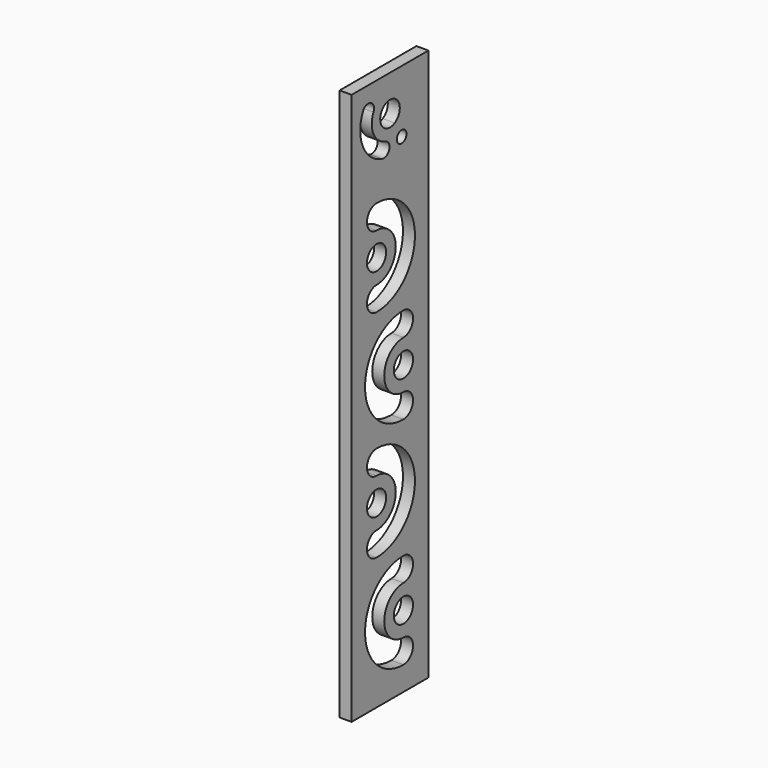
from build123d import *

# Parameters (mm, degrees)
F0_W      = 63.5
F0_H      = 63.5
F0_W_2    = 50.8
F0_H_2    = 50.8
F1_DEPTH  = 165.1
F3_R      = 6.477
F4_DEPTH  = 25.4
F6_DEPTH  = 25.4
F7_R      = 6.35
F8_DEPTH  = 63.501
F9_W      = 145.7979530096
F9_H      = 377.9422044754
F9_W_2    = 50.8
F9_H_2    = 292.1
F10_DEPTH = 63.5
F11_W     = 97.6704657078
F11_H     = 338.8985395432
F12_DEPTH = 57.151


# Not quite as in the source:
# - ends of sketch curves that miss each other by under 0.0002 mm in the source are joined


with BuildPart() as f1:
    # F0 (on Top) → F1 (new body, symmetric)
    with BuildSketch(Plane.XY):
        Rectangle(F0_W, F0_H)
        Rectangle(F0_W_2, F0_H_2, mode=Mode.SUBTRACT)
    extrude(amount=F1_DEPTH, both=True)

    # F3 (on face) → F4 (cut)
    with BuildSketch(Plane.YZ.offset(31.75)):
        with Locations((0, 146.05)):
            Circle(F3_R)
        with BuildLine():
            ThreePointArc((10.1385245046, 129.1766616857), (14.6288058895, 132.8781640138), (17.8406687878, 137.7307595176))
            ThreePointArc((17.8406687878, 137.7307595176), (19.4934269332, 143.3103775076), (19.4426449846, 149.1294124443))
            ThreePointArc((19.4426449846, 149.1294124443), (15.0835370951, 152.2964897102), (11.9164598293, 147.9373818207))
            ThreePointArc((11.9164598293, 147.9373818207), (11.9475842494, 144.3708765369), (10.9346034506, 140.9511106721))
            ThreePointArc((10.9346034506, 140.9511106721), (8.9660423194, 137.9769392343), (6.2139343738, 135.708276517))
            ThreePointArc((6.2139343738, 135.708276517), (4.9104220235, 130.4801740359), (10.1385245046, 129.1766616857))
        make_face()
        with BuildLine():
            ThreePointArc((-10.1385245046, 129.1766616857), (-4.9104220235, 130.4801740359), (-6.2139343738, 135.708276517))
            ThreePointArc((-6.2139343738, 135.708276517), (-8.9660423194, 137.9769392343), (-10.9346034506, 140.9511106721))
            ThreePointArc((-10.9346034506, 140.9511106721), (-11.9475842494, 144.3708765369), (-11.9164598293, 147.9373818207))
            ThreePointArc((-11.9164598293, 147.9373818207), (-15.0835370951, 152.2964897102), (-19.4426449846, 149.1294124443))
            ThreePointArc((-19.4426449846, 149.1294124443), (-19.4934269332, 143.3103775076), (-17.8406687878, 137.7307595176))
            ThreePointArc((-17.8406687878, 137.7307595176), (-14.6288058895, 132.8781640138), (-10.1385245046, 129.1766616857))
        make_face()
    extrude(amount=-F4_DEPTH, mode=Mode.SUBTRACT)

    # F5 (on face) → F6 (cut)
    with BuildSketch(Plane(origin=(-31.75, 0, 0), x_dir=(0, -1, 0), z_dir=(-1, 0, 0))):
        with BuildLine():
            ThreePointArc((-3.1401119103, 140.3850881569), (3.2873259769, 140.4692279278), (6.477, 146.05))
            ThreePointArc((6.477, 146.05), (-3.2873259769, 151.6307720722), (-3.1401119103, 140.3850881569))
        make_face()
        with BuildLine():
            ThreePointArc((-4.5213527214, 132.1654121492), (-4.960680137, 133.7768464516), (-6.1570821771, 134.9423297193))
            ThreePointArc((-6.1570821771, 134.9423297193), (-10.4320253058, 130.5539778468), (-4.5213527214, 132.1654121492))
        make_face()
        with BuildLine():
            ThreePointArc((3.1226517792, 134.3961049058), (0.4285749428, 129.7298269458), (5.0948529028, 127.0357501095))
            ThreePointArc((5.0948529028, 127.0357501095), (17.8406687878, 137.7307595176), (17.8406687878, 154.3692404824))
            ThreePointArc((17.8406687878, 154.3692404824), (12.777460542, 156.2120975737), (10.9346034506, 151.1488893279))
            ThreePointArc((10.9346034506, 151.1488893279), (10.9346034506, 140.9511106721), (3.1226517792, 134.3961049058))
        make_face()
    extrude(amount=-F6_DEPTH, mode=Mode.SUBTRACT)

    # F7 (on face) → F8 (cut, through all)
    with BuildSketch(Plane.YZ.offset(31.75)):
        with BuildLine():
            ThreePointArc((-8.89, 107.949999693), (-15.239999693, 101.6), (-8.89, 95.250000307))
            ThreePointArc((-8.89, 95.250000307), (3.81, 82.55), (-8.89, 69.85))
            ThreePointArc((-8.89, 69.85), (-15.239999693, 63.5), (-8.89, 57.150000307))
            ThreePointArc((-8.89, 57.150000307), (16.509999693, 82.55), (-8.89, 107.949999693))
        make_face()
        with BuildLine():
            ThreePointArc((8.89, 3.07e-07), (15.239999693, 6.35), (8.89, 12.699999693))
            ThreePointArc((8.89, 12.699999693), (-3.81, 25.4), (8.89, 38.1))
            ThreePointArc((8.89, 38.1), (15.24, 44.45), (8.89, 50.8))
            ThreePointArc((8.89, 50.8), (-16.509999693, 25.4), (8.89, 3.07e-07))
        make_face()
        with BuildLine():
            ThreePointArc((-8.89, -6.350000307), (-15.239999693, -12.7), (-8.89, -19.049999693))
            ThreePointArc((-8.89, -19.049999693), (3.81, -31.75), (-8.89, -44.45))
            ThreePointArc((-8.89, -44.45), (-15.239999693, -50.8), (-8.89, -57.149999693))
            ThreePointArc((-8.89, -57.149999693), (16.509999693, -31.75), (-8.89, -6.350000307))
        make_face()
        with BuildLine():
            ThreePointArc((8.89, -114.299999693), (15.239999693, -107.95), (8.89, -101.600000307))
            ThreePointArc((8.89, -101.600000307), (-3.81, -88.9), (8.89, -76.2))
            ThreePointArc((8.89, -76.2), (15.24, -69.85), (8.89, -63.5))
            ThreePointArc((8.89, -63.5), (-16.509999693, -88.9), (8.89, -114.299999693))
        make_face()
        with Locations((-8.89, 82.55)):
            Circle(F7_R)
        with Locations((8.89, 25.4)):
            Circle(F7_R)
        with Locations((8.89, -88.9)):
            Circle(F7_R)
        with Locations((-8.89, -31.75)):
            Circle(F7_R)
    extrude(amount=-F8_DEPTH, mode=Mode.SUBTRACT)

    # F9 (on face) → F10 (cut, symmetric)
    with BuildSketch(Plane(origin=(25.4, 0, 0), x_dir=(0, -1, 0), z_dir=(-1, 0, 0))):
        Rectangle(F9_W, F9_H)
        with Locations((0, 19.05)):
            Rectangle(F9_W_2, F9_H_2, mode=Mode.SUBTRACT)
    extrude(amount=F10_DEPTH, both=True, mode=Mode.SUBTRACT)

    # F11 (on face) → F12 (cut, through all)
    with BuildSketch(Plane.YZ.offset(-25.4)):
        Rectangle(F11_W, F11_H)
    extrude(amount=F12_DEPTH, mode=Mode.SUBTRACT)


solid = f1.part
